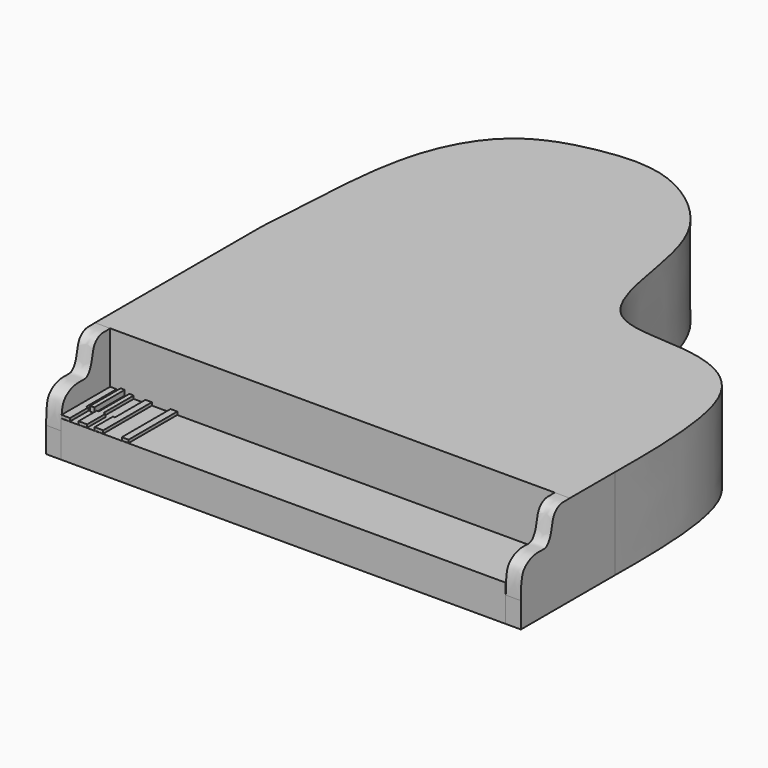
from build123d import *

# Parameters (mm, degrees)
F1_DEPTH  = 13.716
F3_DEPTH  = 2.286
F4_W      = 67.1706
F4_H      = 5.487878
F5_DEPTH  = 9.2456
F7_DEPTH  = 2.286
F9_DEPTH  = 0.4572
F8_W      = 0.629274
F8_H      = 5.748775
F10_DEPTH = 0.762
F8_W_2    = 1.019199
F8_H_2    = 9.20058
F11_DEPTH = 0.4572


# Not quite as in the source:
# - the program builds the solid bodies; features that only make, move or delete a surface that nothing else refers to are left out


with BuildPart() as f1:
    # F0 (on Top) → F1 (new body)
    with BuildSketch(Plane.XY):
        with BuildLine():
            Line((-71.939357, 31.47507), (-71.939357, 0))
            Line((-71.939357, 0), (-0.196673, 0))
            Line((-0.196673, 0), (-0.196673, 8.553878))
            add(Edge.make_bspline(
                [(-71.939357, 31.47507), (-71.280026, 39.645206), (-71.390784, 55.201123), (-64.173221, 68.480197), (-53.431869, 71.872131), (-42.372269, 72.681335), (-31.100324, 63.729452), (-28.973827, 51.961311), (-26.605915, 38.795949), (-16.456892, 38.488386), (-8.644374, 37.739527), (-0.483658, 31.704651), (-0.102318, 17.782523), (-0.196673, 8.553878)],
                knots=[0, 0, 0, 0, 0.125801, 0.220731, 0.303358, 0.387051, 0.479113, 0.569018, 0.656441, 0.731304, 0.803079, 0.876918, 1, 1, 1, 1], degree=3))
        make_face()
    extrude(amount=F1_DEPTH)

    # F2 (on face) → F3 (join)
    with BuildSketch(Plane.YZ.offset(-0.196673)):
        with BuildLine():
            Line((-9.2458, 0), (0, 0))
            Line((0, 0), (0, 13.716))
            add(Edge.make_bspline(
                [(-9.2458, 3.837853), (-9.228357, 5.189316), (-9.200198, 7.371119), (-8.045473, 8.376502), (-7.137937, 8.801358), (-6.235997, 8.964577), (-5.372635, 8.936603), (-4.34019, 8.884541), (-3.64996, 10.039759), (-3.396048, 11.201037), (-3.151884, 12.55509), (-2.574364, 13.273116), (-1.698244, 13.735755), (-0.851194, 13.679409), (-0.284549, 13.703768), (0, 13.716)],
                knots=[0, 0, 0, 0, 0.134349, 0.216892, 0.287386, 0.354969, 0.421952, 0.490827, 0.568998, 0.649168, 0.731874, 0.799493, 0.868612, 0.934022, 1, 1, 1, 1], degree=3))
            Line((-9.2458, 3.837853), (-9.2458, 0))
        make_face()
    extrude(amount=-F3_DEPTH)

    # F4 (on face) → F5 (join)
    with BuildSketch(Plane.XZ):
        with Locations((-36.067973, 2.743939)):
            Rectangle(F4_W, F4_H)
    extrude(amount=F5_DEPTH)

    # F6 (on face) → F7 (join)
    with BuildSketch(Plane(origin=(-69.653273, 0, 0), x_dir=(0, -1, 0), z_dir=(-1, 0, 0))):
        with BuildLine():
            add(Edge.make_bspline(
                [(9.2458, 3.837853), (9.228357, 5.189316), (9.200198, 7.371119), (8.045473, 8.376502), (7.137937, 8.801358), (6.235997, 8.964577), (5.372635, 8.936603), (4.34019, 8.884541), (3.64996, 10.039759), (3.396048, 11.201037), (3.151884, 12.55509), (2.574364, 13.273116), (1.698244, 13.735755), (0.851194, 13.679409), (0.284549, 13.703768), (0, 13.716)],
                knots=[0, 0, 0, 0, 0.134349, 0.216892, 0.287386, 0.354969, 0.421952, 0.490827, 0.568998, 0.649168, 0.731874, 0.799493, 0.868612, 0.934022, 1, 1, 1, 1], degree=3))
            Line((0, 13.716), (0, 0))
            Line((0, 0), (9.2458, 0))
            Line((9.2458, 0), (9.2458, 3.837853))
        make_face()
    extrude(amount=F7_DEPTH)


with BuildPart() as f9:
    # F8 (on face) → F9 (new body)
    with BuildSketch(Plane.XY.offset(5.487878)):
        Polygon((-69.653273, 0), (-69.653273, -9.200579), (-68.361302, -9.200579), (-68.361302, -5.748773), (-68.675939, -5.748773), (-68.675939, 0), align=None)
    extrude(amount=F9_DEPTH)


with BuildPart() as f9b:
    # F8 (on face) → F9, piece 2 (new body)
    with BuildSketch(Plane.XY.offset(5.487878)):
        Polygon((-66.091997, 0), (-66.754693, 0), (-66.754693, -5.748775), (-67.069331, -5.748775), (-67.069331, -9.20058), (-65.77736, -9.20058), (-65.77736, -5.748775), (-66.091997, -5.748775), align=None)
    extrude(amount=F9_DEPTH)


with BuildPart() as f9c:
    # F8 (on face) → F9, piece 3 (new body)
    with BuildSketch(Plane.XY.offset(5.487878)):
        Polygon((-63.342393, 0), (-64.319727, 0), (-64.319727, -5.748775), (-64.634364, -5.748775), (-64.634364, -9.20058), (-63.342393, -9.20058), align=None)
    extrude(amount=F9_DEPTH)


with BuildPart() as f10:
    # F8 (on face) → F10 (new body)
    with BuildSketch(Plane.XY.offset(5.487878)):
        with Locations((-67.767267, -2.874387)):
            Rectangle(F8_W, F8_H)
    extrude(amount=F10_DEPTH)


with BuildPart() as f11:
    # F8 (on face) → F11 (new body)
    with BuildSketch(Plane.XY.offset(5.487878)):
        with Locations((-60.020028, -4.60029)):
            Rectangle(F8_W_2, F8_H_2)
    extrude(amount=F11_DEPTH)


solid = Compound([f1.part, f9.part, f9b.part, f9c.part, f10.part, f11.part])
